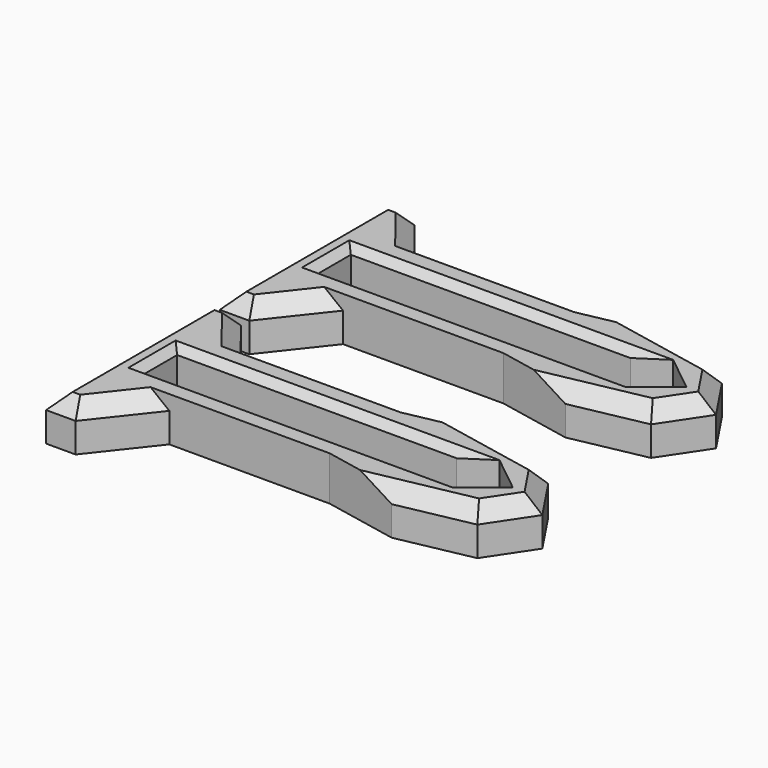
from build123d import *

# Parameters (mm, degrees)
F1_DEPTH = 3
F2_SIZE  = 1
F3_SIZE  = 0.49999


# Not quite as in the source:
# - a fillet or chamfer is up to 0.001 mm smaller than in the source, because OpenCascade refuses the exact size
# - a feature names something its author has since deleted; it is built from what else it names


with BuildPart() as f1:
    # F0 (on Top) → F1 (new body)
    with BuildSketch(Plane.XY):
        Polygon((-13, 9), (-13, -5), (-11, -5), (-7.8552635387, -1), (3, -1), (8, -2), (13, -1), (15, 2), (13, 5), (8, 6), (3, 5), (-7.8552635387, 5), (-11, 9), align=None)
        Polygon((-10.9275523573, 0.5000008065), (-10.9275523573, 2.0000008065), (-10.9275523573, 3.5000008065), (3, 3.5000008065), (8, 3.5000008065), (10.5, 4.0000008065), (13, 2.0000008065), (10.5, 8.065e-07), (8, 0.5000008065), (3, 0.5000008065), align=None, mode=Mode.SUBTRACT)
    extrude(amount=F1_DEPTH)

    # F2
    f2_edges = [f1.edges().sort_by_distance(p)[0] for p in [
        (-12, -5, 3),
        (-13, 2, 3),
        (-12, 9, 3),
        (-9.427632, 7, 3),
        (14, 3.5, 3),
        (14, 0.5, 3),
        (-9.427632, -3, 3),
        (10.5, 5.5, 3),
        (10.5, -1.5, 3),
    ]]
    chamfer(f2_edges, length=F2_SIZE)

    # F3 (size 0.5 in the source; OpenCascade refuses exactly that, so slightly less here)
    f3_edges = [f1.edges().sort_by_distance(p)[0] for p in [
        (-1.463776, 3.500001, 3),
        (-1.463776, 0.500001, 3),
        (-10.927552, 2.000001, 3),
    ]]
    chamfer(f3_edges, length=F3_SIZE)


with BuildPart() as f4_1:
    # F4: copy of F1
    add(f1.part.moved(Location((0, -14.7, 0))))


solid = Compound([f1.part, f4_1.part])
